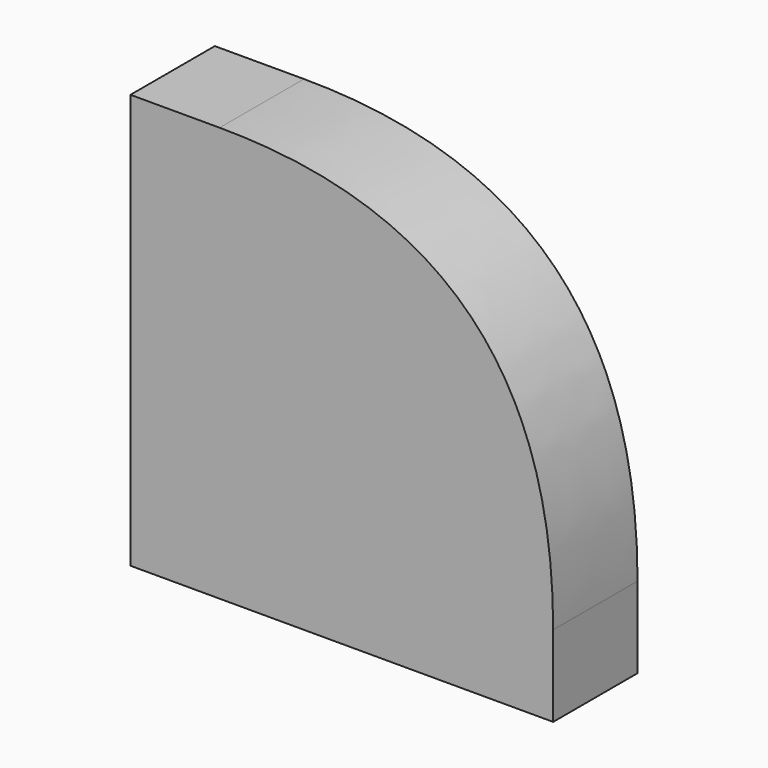
from build123d import *

# Parameters (mm, degrees)
F0_W        = 101.8087677658
F0_H        = 99.8602770269
F1_DEPTH    = 25.4
F2_T1_DEPTH = 427.052710372


# Not quite as in the source:
# - a fillet or chamfer that OpenCascade refuses, or shapes differently, is made with other operations: its cross-section is extruded or revolved along the edge and cut away or added


with BuildPart() as f1:
    # F0 (on Front) → F1 (new body)
    with BuildSketch(Plane.XZ):
        with Locations((-2.1920558065, -5.4801348597)):
            Rectangle(F0_W, F0_H)
    extrude(amount=F1_DEPTH)

    # F2: fillet of radius 80.3305420744 on 1 edges, made by hand

    # F2_s2 → F2_t1 (cut)
    with BuildSketch(Plane.XZ.offset(-200.826355186)):
        with BuildLine():
            add(Edge.make_bspline(
                [(-31.618213998, 44.4500036538), (48.7123280764, 44.4500036538), (48.7123280764, -35.8805384206)],
                knots=[0, 0, 0, 1, 1, 1], degree=2, weights=[1, 1, 1]))
            Line((48.7123280764, -35.8805384206), (48.7123280764, 44.4500036538))
            Line((48.7123280764, 44.4500036538), (-31.618213998, 44.4500036538))
        make_face()
    extrude(amount=F2_T1_DEPTH, mode=Mode.SUBTRACT)


solid = f1.part
